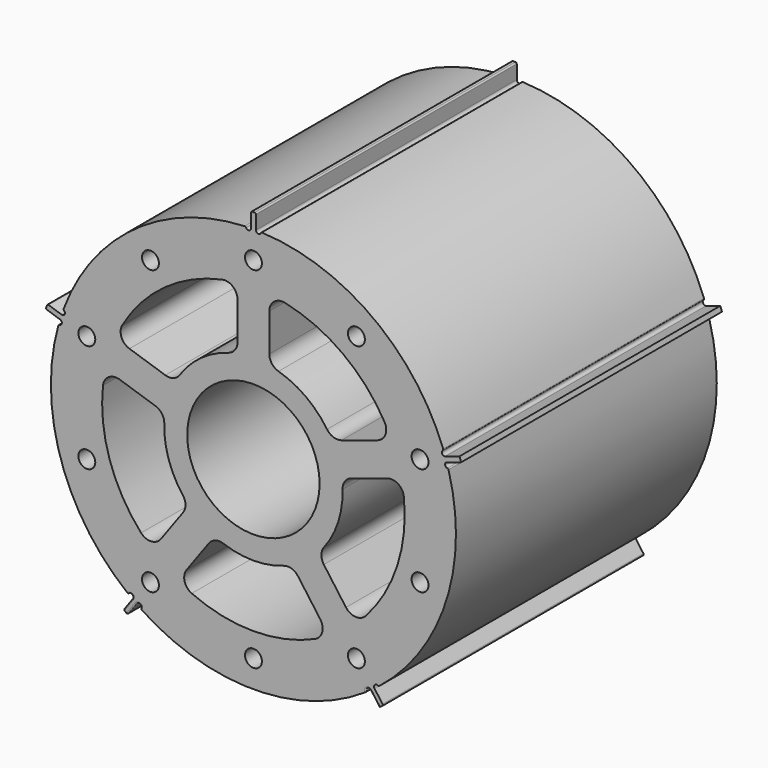
from build123d import *

# Parameters (mm, degrees)
F1_DEPTH = 129.9972
F2_R     = 26.3906
F3_DEPTH = 129.9972
F5_R     = 1.016
F6_DEPTH = 129.9982
F7_R     = 0.508
F9_DEPTH = 129.9982001
F10_R    = 5.08
F12_D    = 6.7564


with BuildPart() as f1:
    # F0 (on Front) → F1 (new body)
    with BuildSketch(Plane.XZ):
        with BuildLine():
            Line((-1.000252, 86.7377727848), (-1.000252, 80.7429446248))
            ThreePointArc((-1.000252, 80.7429446248), (-47.4631536273, 65.3274265412), (-76.4820087636, 25.9022382475))
            Line((-76.4820087636, 25.9022382475), (-82.1834291493, 27.7547420273))
            Line((-82.1834291493, 27.7547420273), (-82.8016188826, 25.8521496622))
            Line((-82.8016188826, 25.8521496622), (-77.1001984969, 23.9996458824))
            ThreePointArc((-77.1001984969, 23.9996458824), (-76.7969957822, -24.9528565412), (-48.2687329438, -64.7344810031))
            Line((-48.2687329438, -64.7344810031), (-51.7924045263, -69.584398863))
            Line((-51.7924045263, -69.584398863), (-50.1739627929, -70.7602656113))
            Line((-50.1739627929, -70.7602656113), (-46.6502912104, -65.9103477515))
            ThreePointArc((-46.6502912104, -65.9103477515), (0, -80.74914), (46.6502912104, -65.9103477515))
            ThreePointArc((46.6502912104, -65.9103477515), (47.4631536273, -65.3274265412), (48.2687329438, -64.7344810031))
            ThreePointArc((48.2687329438, -64.7344810031), (76.7969957822, -24.9528565412), (77.1001984969, 23.9996458824))
            Line((77.1001984969, 23.9996458824), (82.8016188826, 25.8521496622))
            Line((82.8016188826, 25.8521496622), (82.1834291493, 27.7547420273))
            Line((82.1834291493, 27.7547420273), (76.4820087636, 25.9022382475))
            ThreePointArc((76.4820087636, 25.9022382475), (47.4631536273, 65.3274265412), (1.000252, 80.7429446248))
            Line((1.000252, 80.7429446248), (1.000252, 86.7377727848))
            Line((1.000252, 86.7377727848), (-1.000252, 86.7377727848))
        make_face()
        with BuildLine():
            Line((51.7924045263, -69.584398863), (48.2687329438, -64.7344810031))
            ThreePointArc((48.2687329438, -64.7344810031), (47.4631536273, -65.3274265412), (46.6502912104, -65.9103477515))
            Line((46.6502912104, -65.9103477515), (50.1739627929, -70.7602656113))
            Line((50.1739627929, -70.7602656113), (51.7924045263, -69.584398863))
        make_face()
    extrude(amount=F1_DEPTH)

    # F2 (on Front) → F3 (cut, through all)
    with BuildSketch(Plane.XZ):
        Circle(F2_R)
    extrude(amount=F3_DEPTH, mode=Mode.SUBTRACT)

    # F5 (on face) → F6 (cut, through all)
    with BuildSketch(Plane(origin=(0, 0, 0), x_dir=(-1, 0, 0), z_dir=(0, 1, 0))):
        with Locations((-2.016252, 80.7429446248)):
            Circle(F5_R)
        with Locations((2.016252, 80.7429446248)):
            Circle(F5_R)
        with Locations((-76.1680474973, 26.868511668)):
            Circle(F5_R)
        with Locations((-77.4141597632, 23.0333724618)):
            Circle(F5_R)
        with Locations((-49.09069421, -64.1372911868)):
            Circle(F5_R)
        with Locations((-45.8283299442, -66.5075375678)):
            Circle(F5_R)
        with Locations((45.8283299442, -66.5075375678)):
            Circle(F5_R)
        with Locations((49.09069421, -64.1372911868)):
            Circle(F5_R)
        with Locations((77.4141597632, 23.0333724618)):
            Circle(F5_R)
        with Locations((76.1680474973, 26.868511668)):
            Circle(F5_R)
    extrude(amount=-F6_DEPTH, mode=Mode.SUBTRACT)

    # F7
    f7_edges = [f1.edges().sort_by_distance(p)[0] for p in [
        (-1.000252, -64.9986, 86.737773),
        (1.000252, -64.9986, 86.737773),
        (-3.030986, -64.9986, 80.692235),
        (3.030986, -64.9986, 80.692235),
        (-82.183429, -64.9986, 27.754742),
        (-82.801619, -64.9986, 25.85215),
        (-51.792405, -64.9986, -69.584399),
        (-50.173963, -64.9986, -70.760266),
        (49.881824, -64.9986, -63.49982),
        (77.679502, -64.9986, 22.052633),
        (50.173963, -64.9986, -70.760266),
        (51.792405, -64.9986, -69.584399),
        (75.80625, -64.9986, 27.817911),
        (-48.473171, -129.9972, -63.330494),
        (-50.030569, -129.9972, -67.15944),
        (-48.412127, -129.9972, -68.335307),
        (-45.251845, -129.9972, -65.670925),
        (45.251845, -129.9972, -65.670925),
        (48.412127, -129.9972, -68.335307),
        (44.977587, -64.9986, -67.062958),
        (-44.977587, -64.9986, -67.062958),
        (-49.881824, -64.9986, -63.49982),
        (-77.679502, -64.9986, 22.052633),
        (-75.80625, -64.9986, 27.817911),
    ]]
    fillet(f7_edges, radius=F7_R)

    # F8 (on face) → F9 (cut, through all)
    with BuildSketch(Plane(origin=(0, 0, 0), x_dir=(-1, 0, 0), z_dir=(0, 1, 0))):
        with BuildLine():
            Line((-6.35, 34.9884423774), (-6.35, 59.9898585179))
            ThreePointArc((-6.35, 59.9898585179), (-35.4581453445, 48.8039501857), (-55.0914879408, 24.5770946507))
            Line((-55.0914879408, 24.5770946507), (-31.3137282038, 16.8512321798))
            ThreePointArc((-31.3137282038, 16.8512321798), (-20.9016435715, 28.76864432), (-6.35, 34.9884423774))
        make_face()
        with BuildLine():
            ThreePointArc((55.0914879408, 24.5770946507), (35.4581453445, 48.8039501857), (6.35, 59.9898585179))
            Line((6.35, 59.9898585179), (6.35, 34.9884423774))
            ThreePointArc((6.35, 34.9884423774), (20.9016435715, 28.76864432), (31.3137282038, 16.8512321798))
            Line((31.3137282038, 16.8512321798), (55.0914879408, 24.5770946507))
        make_face()
        with BuildLine():
            Line((25.7029483444, -24.573808138), (40.3984120382, -44.8003786791))
            ThreePointArc((40.3984120382, -44.8003786791), (57.3724843455, -18.6414501857), (59.0160037694, 12.4986768937))
            Line((59.0160037694, 12.4986768937), (35.2382440324, 4.7728144229))
            ThreePointArc((35.2382440324, 4.7728144229), (33.8195697195, -10.98864432), (25.7029483444, -24.573808138))
        make_face()
        with BuildLine():
            Line((-15.4284325159, -32.0386808421), (-30.1238962097, -52.2652513832))
            ThreePointArc((-30.1238962097, -52.2652513832), (0, -60.325), (30.1238962097, -52.2652513832))
            Line((30.1238962097, -52.2652513832), (15.4284325159, -32.0386808421))
            ThreePointArc((15.4284325159, -32.0386808421), (0, -35.56), (-15.4284325159, -32.0386808421))
        make_face()
        with BuildLine():
            Line((-35.2382440324, 4.7728144229), (-59.0160037694, 12.4986768937))
            ThreePointArc((-59.0160037694, 12.4986768937), (-57.3724843455, -18.6414501857), (-40.3984120382, -44.8003786791))
            Line((-40.3984120382, -44.8003786791), (-25.7029483444, -24.573808138))
            ThreePointArc((-25.7029483444, -24.573808138), (-33.8195697195, -10.98864432), (-35.2382440324, 4.7728144229))
        make_face()
    extrude(amount=-F9_DEPTH, mode=Mode.SUBTRACT)

    # F10
    f10_edges = [f1.edges().sort_by_distance(p)[0] for p in [
        (55.091488, -64.9986, 24.577095),
        (31.313728, -64.9986, 16.851232),
        (6.35, -64.9986, 34.988442),
        (6.35, -64.9986, 59.989859),
        (-55.091488, -64.9986, 24.577095),
        (-31.313728, -64.9986, 16.851232),
        (-6.35, -64.9986, 34.988442),
        (-6.35, -64.9986, 59.989859),
        (-59.016004, -64.9986, 12.498677),
        (-40.398412, -64.9986, -44.800379),
        (-25.702948, -64.9986, -24.573808),
        (-35.238244, -64.9986, 4.772814),
        (30.123896, -64.9986, -52.265251),
        (-30.123896, -64.9986, -52.265251),
        (-15.428433, -64.9986, -32.038681),
        (15.428433, -64.9986, -32.038681),
        (35.238244, -64.9986, 4.772814),
        (25.702948, -64.9986, -24.573808),
        (40.398412, -64.9986, -44.800379),
        (59.016004, -64.9986, 12.498677),
    ]]
    fillet(f10_edges, radius=F10_R)

    # F12 (through all)
    with Locations(Plane(origin=(0, 0, 0), x_dir=(-1, 0, 0), z_dir=(0, 1, 0))):
        with Locations((0, 69.85), (-41.0567998726, 56.5098370571), (-66.4312976632, 21.5848370571), (-66.4312976632, -21.5848370571), (-41.0567998726, -56.5098370571), (0, -69.85), (41.0567998726, -56.5098370571), (66.4312976632, -21.5848370571), (66.4312976632, 21.5848370571), (41.0567998726, 56.5098370571)):
            Hole(F12_D / 2)


solid = f1.part
